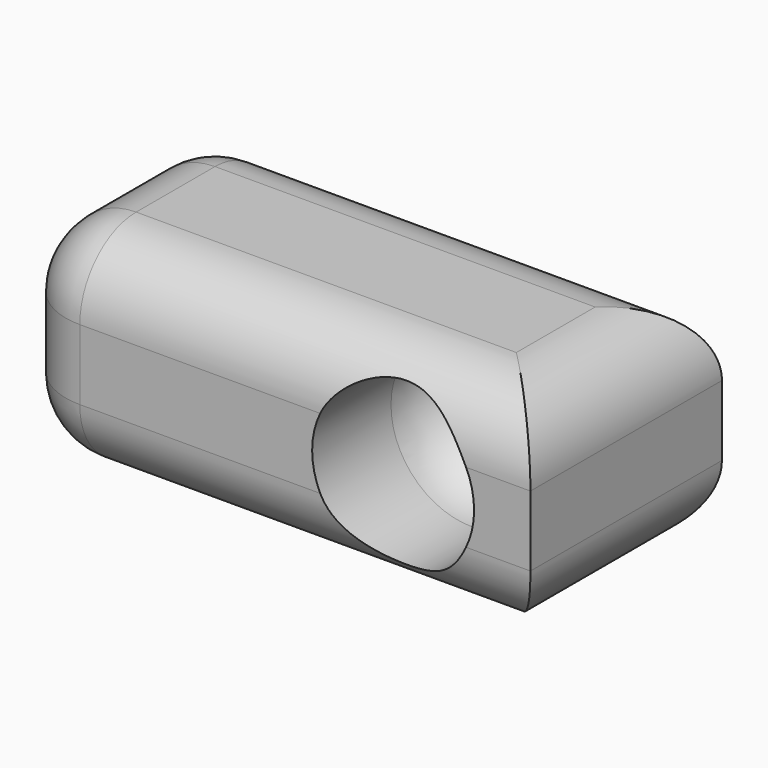
from build123d import *

# Parameters (mm, degrees)
F0_W         = 37
F0_H         = 15
F1_DEPTH     = 17
F2_R         = 5.75
F3_DEPTH     = 7
F6_T1_DEPTH  = 44.5
F6_T3_DEPTH  = 42
F6_T5_DEPTH  = 7
F6_T7_DEPTH  = 5
F6_S11_W     = 5
F6_S11_H     = 5
F6_T12_DEPTH = 5
F6_S17_W     = 5
F6_S17_H     = 5
F6_T18_DEPTH = 5
F6_S23_W     = 5
F6_S23_H     = 5
F6_T24_DEPTH = 5
F6_S29_W     = 5
F6_S29_H     = 5
F6_T30_DEPTH = 5


# Not quite as in the source:
# - a fillet or chamfer that OpenCascade refuses, or shapes differently, is made with other operations: its cross-section is extruded or revolved along the edge and cut away or added


with BuildPart() as f1:
    # F0 (on Front) → F1 (new body)
    with BuildSketch(Plane.XZ):
        Rectangle(F0_W, F0_H)
    extrude(amount=F1_DEPTH)

    # F2 (on face) → F3 (cut)
    with BuildSketch(Plane.XZ.offset(17)):
        with Locations((8.75, 0)):
            Circle(F2_R)
    extrude(amount=-F3_DEPTH, mode=Mode.SUBTRACT)

    # F4 (on face) → F5 (revolve, cut)
    with BuildSketch(Plane.XZ.offset(10)):
        with BuildLine():
            Line((8.75, 0), (8.75, 5.75))
            ThreePointArc((8.75, 5.75), (3, 0), (8.75, -5.75))
            Line((8.75, -5.75), (8.75, 0))
        make_face()
    revolve(axis=Axis((8.75, -10, 2.875), (0, 0, 1)), mode=Mode.SUBTRACT)

    # F6: fillet of radius 5 on 10 edges, made by hand

    # F6_s2 → F6_t1 (cut)
    with BuildSketch(Plane.YZ.offset(-13.5)):
        with BuildLine():
            ThreePointArc((-17, 2.5), (-15.5355339059, 6.0355339059), (-12, 7.5))
            Line((-12, 7.5), (-17, 7.5))
            Line((-17, 7.5), (-17, 2.5))
        make_face()
        with BuildLine():
            ThreePointArc((-12, -7.5), (-15.5355339059, -6.0355339059), (-17, -2.5))
            Line((-17, -2.5), (-17, -7.5))
            Line((-17, -7.5), (-12, -7.5))
        make_face()
        with BuildLine():
            ThreePointArc((0, 2.5), (-1.4644660941, 6.0355339059), (-5, 7.5))
            Line((-5, 7.5), (0, 7.5))
            Line((0, 7.5), (0, 2.5))
        make_face()
        with BuildLine():
            ThreePointArc((-5, -7.5), (-1.4644660941, -6.0355339059), (0, -2.5))
            Line((0, -2.5), (0, -7.5))
            Line((0, -7.5), (-5, -7.5))
        make_face()
    extrude(amount=F6_T1_DEPTH, mode=Mode.SUBTRACT)

    # F6_s4 → F6_t3 (cut)
    with BuildSketch(Plane.XZ.offset(-12.5)):
        with BuildLine():
            ThreePointArc((18.5, 2.5), (17.0355339059, 6.0355339059), (13.5, 7.5))
            Line((13.5, 7.5), (18.5, 7.5))
            Line((18.5, 7.5), (18.5, 2.5))
        make_face()
        with BuildLine():
            ThreePointArc((13.5, -7.5), (17.0355339059, -6.0355339059), (18.5, -2.5))
            Line((18.5, -2.5), (18.5, -7.5))
            Line((18.5, -7.5), (13.5, -7.5))
        make_face()
    extrude(amount=F6_T3_DEPTH, mode=Mode.SUBTRACT)

    # F6_s6 → F6_t5 (cut)
    with BuildSketch(Plane.XZ.offset(5)):
        with BuildLine():
            ThreePointArc((-18.5, 2.5), (-17.0355339059, 6.0355339059), (-13.5, 7.5))
            Line((-13.5, 7.5), (-18.5, 7.5))
            Line((-18.5, 7.5), (-18.5, 2.5))
        make_face()
        with BuildLine():
            ThreePointArc((-13.5, -7.5), (-17.0355339059, -6.0355339059), (-18.5, -2.5))
            Line((-18.5, -2.5), (-18.5, -7.5))
            Line((-18.5, -7.5), (-13.5, -7.5))
        make_face()
    extrude(amount=F6_T5_DEPTH, mode=Mode.SUBTRACT)

    # F6_s8 → F6_t7 (cut)
    with BuildSketch(Plane.XY.offset(-2.5)):
        with BuildLine():
            ThreePointArc((-18.5, -12), (-17.0355339059, -15.5355339059), (-13.5, -17))
            Line((-13.5, -17), (-18.5, -17))
            Line((-18.5, -17), (-18.5, -12))
        make_face()
        with BuildLine():
            ThreePointArc((-18.5, -5), (-17.0355339059, -1.4644660941), (-13.5, 0))
            Line((-13.5, 0), (-18.5, 0))
            Line((-18.5, 0), (-18.5, -5))
        make_face()
    extrude(amount=F6_T7_DEPTH, mode=Mode.SUBTRACT)


with BuildPart() as f6_tool10:
    # F6_s11 → F6_t12 (new body)
    with BuildSketch(Plane.YZ.offset(-13.5)):
        with Locations((-14.5, 5)):
            Rectangle(F6_S11_W, F6_S11_H)
    extrude(amount=-F6_T12_DEPTH)

    # F6_s13 → F6_t14 (revolve, cut)
    with BuildSketch(Plane(origin=(-13.5, -12, 2.5), x_dir=(0, 0.7071067812, -0.7071067812), z_dir=(0, 0.7071067812, 0.7071067812))):
        with BuildLine():
            ThreePointArc((0, -5), (5, 0), (0, 5))
            Line((0, 5), (0, -5))
        make_face()
    revolve(axis=Axis((-13.5, -12, 2.5), (-1, 0, 0)), mode=Mode.SUBTRACT)


with BuildPart() as f1_1:
    add(f1.part)

    # F6_t9: cut F6_tool10
    add(f6_tool10.part, mode=Mode.SUBTRACT)


with BuildPart() as f6_tool16:
    # F6_s17 → F6_t18 (new body)
    with BuildSketch(Plane.XY.offset(-2.5)):
        with Locations((-16, -14.5)):
            Rectangle(F6_S17_W, F6_S17_H)
    extrude(amount=-F6_T18_DEPTH)

    # F6_s19 → F6_t20 (revolve, cut)
    with BuildSketch(Plane(origin=(-13.5, -12, -2.5), x_dir=(0.7071067812, 0.7071067812, 0), z_dir=(-0.7071067812, 0.7071067812, 0))):
        with BuildLine():
            ThreePointArc((0, -5), (5, 0), (0, 5))
            Line((0, 5), (0, -5))
        make_face()
    revolve(axis=Axis((-13.5, -12, -2.5), (0, 0, -1)), mode=Mode.SUBTRACT)


with BuildPart() as f1_2:
    add(f1_1.part)

    # F6_t15: cut F6_tool16
    add(f6_tool16.part, mode=Mode.SUBTRACT)


with BuildPart() as f6_tool22:
    # F6_s23 → F6_t24 (new body)
    with BuildSketch(Plane.YZ.offset(-13.5)):
        with Locations((-2.5, 5)):
            Rectangle(F6_S23_W, F6_S23_H)
    extrude(amount=-F6_T24_DEPTH)

    # F6_s25 → F6_t26 (revolve, cut)
    with BuildSketch(Plane(origin=(-13.5, -5, 2.5), x_dir=(0, -0.7071067812, -0.7071067812), z_dir=(0, 0.7071067812, -0.7071067812))):
        with BuildLine():
            ThreePointArc((0, -5), (5, 0), (0, 5))
            Line((0, 5), (0, -5))
        make_face()
    revolve(axis=Axis((-13.5, -5, 2.5), (-1, 0, 0)), mode=Mode.SUBTRACT)


with BuildPart() as f1_3:
    add(f1_2.part)

    # F6_t21: cut F6_tool22
    add(f6_tool22.part, mode=Mode.SUBTRACT)


with BuildPart() as f6_tool28:
    # F6_s29 → F6_t30 (new body)
    with BuildSketch(Plane.XY.offset(-2.5)):
        with Locations((-16, -2.5)):
            Rectangle(F6_S29_W, F6_S29_H)
    extrude(amount=-F6_T30_DEPTH)

    # F6_s31 → F6_t32 (revolve, cut)
    with BuildSketch(Plane(origin=(-13.5, -5, -2.5), x_dir=(0.7071067812, -0.7071067812, 0), z_dir=(0.7071067812, 0.7071067812, 0))):
        with BuildLine():
            ThreePointArc((0, -5), (5, 0), (0, 5))
            Line((0, 5), (0, -5))
        make_face()
    revolve(axis=Axis((-13.5, -5, -2.5), (0, 0, -1)), mode=Mode.SUBTRACT)


with BuildPart() as f1_4:
    add(f1_3.part)

    # F6_t27: cut F6_tool28
    add(f6_tool28.part, mode=Mode.SUBTRACT)


solid = f1_4.part
